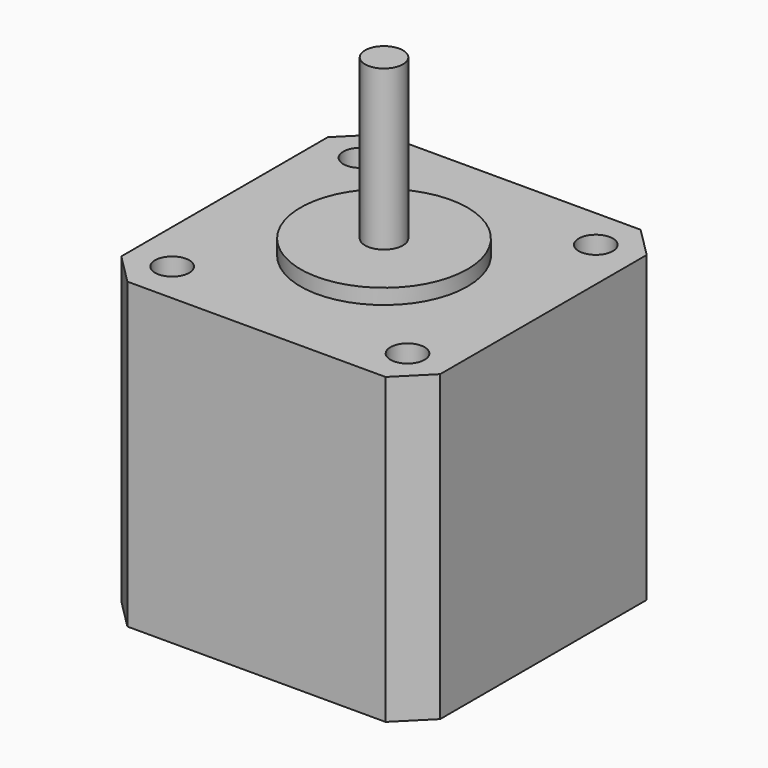
from build123d import *

# Parameters (mm, degrees)
F1_W            = 42
F1_H            = 42
F2_DEPTH        = 40
F3_R            = 11
F4_DEPTH        = 2
F5_R            = 2.5
F6_DEPTH        = 21
F8_D            = 4.5
F8_COPIES_COUNT = 4
F9_SIZE         = 4


# Not quite as in the source:
# - a pattern or mirror of a feature is missing from the dataset's text; its kind, count and spacing are read off the source's solid


with BuildPart() as f2:
    # F1 (on Top) → F2 (new body)
    with BuildSketch(Plane.XY):
        Rectangle(F1_W, F1_H)
    extrude(amount=F2_DEPTH)

    # F3 (on face) → F4 (join)
    with BuildSketch(Plane.XY.offset(40)):
        Circle(F3_R)
    extrude(amount=F4_DEPTH)

    # F5 (on face) → F6 (join)
    with BuildSketch(Plane.XY.offset(42)):
        Circle(F5_R)
    extrude(amount=F6_DEPTH)

    # F8 (through all)
    with Locations(Plane.XY.offset(40)):
        with Locations((15.5, 15.5)):
            f8 = Hole(F8_D / 2)

    # F8_copies: F8 ×4 about axis
    f8_copies_axis = Axis((0, 0, 0), (0, 0, 1))
    for i in range(1, F8_COPIES_COUNT):
        add(f8.rotate(f8_copies_axis, i * 360 / F8_COPIES_COUNT), mode=Mode.SUBTRACT)

    # F9
    f9_edges = [f2.edges().sort_by_distance(p)[0] for p in [
        (21, 21, 20),
        (21, -21, 20),
        (-21, -21, 20),
        (-21, 21, 20),
    ]]
    chamfer(f9_edges, length=F9_SIZE)


solid = f2.part
